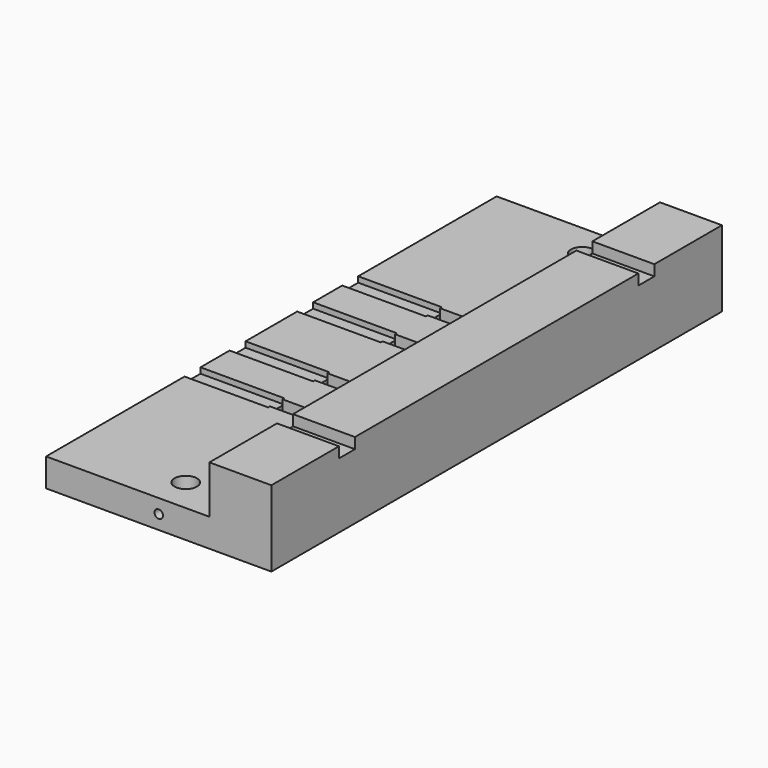
from build123d import *

# Parameters (mm, degrees)
F0_W     = 22
F0_H     = 30
F0_R     = 4
F0_R_2   = 1.5
F0_H_2   = 7.1
F0_H_3   = 125.8
F0_R_3   = 1.8
F1_DEPTH = 10
F2_DEPTH = 4.5
F3_DEPTH = 17
F4_DEPTH = 13.2
F5_R     = 1.5
F6_DEPTH = 15
F7_R     = 1.5
F8_DEPTH = 15
F9_DEPTH = 2


# Not quite as in the source:
# - a feature names something its author has since deleted; it is built from what else it names


with BuildPart() as f1:
    # F0 (on Top) → F1 (new body)
    with BuildSketch(Plane.XY):
        with Locations((29, -85)):
            Rectangle(F0_W, F0_H)
        with BuildLine():
            Line((-40, -100), (18, -100))
            Line((18, -100), (18, -70))
            Line((18, -70), (18, -62.9))
            Line((18, -62.9), (18, 62.9))
            Line((18, 62.9), (18, 70))
            Line((18, 70), (18, 100))
            Line((18, 100), (-40, 100))
            Line((-40, 100), (-40, 38.55))
            Line((-40, 38.55), (-10.3232520311, 38.55))
            Line((-10.3232520311, 38.55), (-10.3232520311, 37.75))
            Line((-10.3232520311, 37.75), (-2.3232520311, 37.75))
            ThreePointArc((-2.3232520311, 37.75), (3.6, 35), (-2.3232520311, 32.25))
            Line((-2.3232520311, 32.25), (-10.3232520311, 32.25))
            Line((-10.3232520311, 32.25), (-10.3232520311, 31.45))
            Line((-10.3232520311, 31.45), (-40, 31.45))
            Line((-40, 31.45), (-40, 18.55))
            Line((-40, 18.55), (-10.3232520311, 18.55))
            Line((-10.3232520311, 18.55), (-10.3232520311, 17.75))
            Line((-10.3232520311, 17.75), (-2.3232520311, 17.75))
            ThreePointArc((-2.3232520311, 17.75), (3.6, 15), (-2.3232520311, 12.25))
            Line((-2.3232520311, 12.25), (-10.3232520311, 12.25))
            Line((-10.3232520311, 12.25), (-10.3232520311, 11.45))
            Line((-10.3232520311, 11.45), (-40, 11.45))
            Line((-40, 11.45), (-40, -11.45))
            Line((-40, -11.45), (-10.3232520311, -11.45))
            Line((-10.3232520311, -11.45), (-10.3232520311, -12.25))
            Line((-10.3232520311, -12.25), (-2.3232520311, -12.25))
            ThreePointArc((-2.3232520311, -12.25), (3.6, -15), (-2.3232520311, -17.75))
            Line((-2.3232520311, -17.75), (-10.3232520311, -17.75))
            Line((-10.3232520311, -17.75), (-10.3232520311, -18.55))
            Line((-10.3232520311, -18.55), (-40, -18.55))
            Line((-40, -18.55), (-40, -31.45))
            Line((-40, -31.45), (-10.3232520311, -31.45))
            Line((-10.3232520311, -31.45), (-10.3232520311, -32.25))
            Line((-10.3232520311, -32.25), (-2.3232520311, -32.25))
            ThreePointArc((-2.3232520311, -32.25), (3.6, -35), (-2.3232520311, -37.75))
            Line((-2.3232520311, -37.75), (-10.3232520311, -37.75))
            Line((-10.3232520311, -37.75), (-10.3232520311, -38.55))
            Line((-10.3232520311, -38.55), (-40, -38.55))
            Line((-40, -38.55), (-40, -100))
        make_face()
        with Locations((0, -88)):
            Circle(F0_R, mode=Mode.SUBTRACT)
        with Locations((0, -66.45)):
            Circle(F0_R_2, mode=Mode.SUBTRACT)
        with Locations((0, 66.45)):
            Circle(F0_R_2, mode=Mode.SUBTRACT)
        with Locations((0, 88)):
            Circle(F0_R, mode=Mode.SUBTRACT)
        with Locations((29, -66.45)):
            Rectangle(F0_W, F0_H_2)
        with Locations((29, 0)):
            Rectangle(F0_W, F0_H_3)
        Polygon((-40, -31.45), (-40, -38.55), (-10.3232520311, -38.55), (-10.3232520311, -37.75), (-10.3232520311, -32.25), (-10.3232520311, -31.45), align=None)
        with Locations((29, 66.45)):
            Rectangle(F0_W, F0_H_2)
        with Locations((29, 85)):
            Rectangle(F0_W, F0_H)
        Polygon((-40, -11.45), (-40, -18.55), (-10.3232520311, -18.55), (-10.3232520311, -17.75), (-10.3232520311, -12.25), (-10.3232520311, -11.45), align=None)
        Polygon((-40, 18.55), (-40, 11.45), (-10.3232520311, 11.45), (-10.3232520311, 12.25), (-10.3232520311, 17.75), (-10.3232520311, 18.55), align=None)
        Polygon((-10.3232520311, 38.55), (-40, 38.55), (-40, 31.45), (-10.3232520311, 31.45), (-10.3232520311, 32.25), (-10.3232520311, 37.75), align=None)
        with BuildLine():
            Line((-10.3232520311, 17.75), (-10.3232520311, 12.25))
            Line((-10.3232520311, 12.25), (-2.3232520311, 12.25))
            ThreePointArc((-2.3232520311, 12.25), (3.6, 15), (-2.3232520311, 17.75))
            Line((-2.3232520311, 17.75), (-10.3232520311, 17.75))
        make_face()
        with Locations((0, 15)):
            Circle(F0_R_3, mode=Mode.SUBTRACT)
        with BuildLine():
            Line((-2.3232520311, 37.75), (-10.3232520311, 37.75))
            Line((-10.3232520311, 37.75), (-10.3232520311, 32.25))
            Line((-10.3232520311, 32.25), (-2.3232520311, 32.25))
            ThreePointArc((-2.3232520311, 32.25), (3.6, 35), (-2.3232520311, 37.75))
        make_face()
        with Locations((0, 35)):
            Circle(F0_R_3, mode=Mode.SUBTRACT)
        with BuildLine():
            Line((-10.3232520311, -12.25), (-10.3232520311, -17.75))
            Line((-10.3232520311, -17.75), (-2.3232520311, -17.75))
            ThreePointArc((-2.3232520311, -17.75), (3.6, -15), (-2.3232520311, -12.25))
            Line((-2.3232520311, -12.25), (-10.3232520311, -12.25))
        make_face()
        with Locations((0, -15)):
            Circle(F0_R_3, mode=Mode.SUBTRACT)
        with BuildLine():
            Line((-10.3232520311, -32.25), (-10.3232520311, -37.75))
            Line((-10.3232520311, -37.75), (-2.3232520311, -37.75))
            ThreePointArc((-2.3232520311, -37.75), (3.6, -35), (-2.3232520311, -32.25))
            Line((-2.3232520311, -32.25), (-10.3232520311, -32.25))
        make_face()
        with Locations((0, -35)):
            Circle(F0_R_3, mode=Mode.SUBTRACT)
    extrude(amount=-F1_DEPTH)

    # F0 (on Top) → F2 (cut)
    with BuildSketch(Plane.XY):
        with BuildLine():
            Line((-10.3232520311, -32.25), (-10.3232520311, -37.75))
            Line((-10.3232520311, -37.75), (-2.3232520311, -37.75))
            ThreePointArc((-2.3232520311, -37.75), (3.6, -35), (-2.3232520311, -32.25))
            Line((-2.3232520311, -32.25), (-10.3232520311, -32.25))
        make_face()
        with Locations((0, -35)):
            Circle(F0_R_3, mode=Mode.SUBTRACT)
        with BuildLine():
            Line((-10.3232520311, -12.25), (-10.3232520311, -17.75))
            Line((-10.3232520311, -17.75), (-2.3232520311, -17.75))
            ThreePointArc((-2.3232520311, -17.75), (3.6, -15), (-2.3232520311, -12.25))
            Line((-2.3232520311, -12.25), (-10.3232520311, -12.25))
        make_face()
        with Locations((0, -15)):
            Circle(F0_R_3, mode=Mode.SUBTRACT)
        with BuildLine():
            Line((-10.3232520311, 17.75), (-10.3232520311, 12.25))
            Line((-10.3232520311, 12.25), (-2.3232520311, 12.25))
            ThreePointArc((-2.3232520311, 12.25), (3.6, 15), (-2.3232520311, 17.75))
            Line((-2.3232520311, 17.75), (-10.3232520311, 17.75))
        make_face()
        with Locations((0, 15)):
            Circle(F0_R_3, mode=Mode.SUBTRACT)
        with BuildLine():
            Line((-2.3232520311, 37.75), (-10.3232520311, 37.75))
            Line((-10.3232520311, 37.75), (-10.3232520311, 32.25))
            Line((-10.3232520311, 32.25), (-2.3232520311, 32.25))
            ThreePointArc((-2.3232520311, 32.25), (3.6, 35), (-2.3232520311, 37.75))
        make_face()
        with Locations((0, 35)):
            Circle(F0_R_3, mode=Mode.SUBTRACT)
    extrude(amount=-F2_DEPTH, mode=Mode.SUBTRACT)

    # F0 (on Top) → F3 (join)
    with BuildSketch(Plane.XY):
        with Locations((29, -85)):
            Rectangle(F0_W, F0_H)
        with Locations((29, 85)):
            Rectangle(F0_W, F0_H)
        with Locations((29, 0)):
            Rectangle(F0_W, F0_H_3)
    extrude(amount=F3_DEPTH)

    # F0 (on Top) → F4 (join)
    with BuildSketch(Plane.XY):
        with Locations((29, 66.45)):
            Rectangle(F0_W, F0_H_2)
        with Locations((29, -66.45)):
            Rectangle(F0_W, F0_H_2)
    extrude(amount=F4_DEPTH)

    # F5 (on face) → F6 (cut)
    with BuildSketch(Plane(origin=(0, 100, 0), x_dir=(-1, 0, 0), z_dir=(0, 1, 0))):
        with Locations((0, -5)):
            Circle(F5_R)
    extrude(amount=-F6_DEPTH, mode=Mode.SUBTRACT)

    # F7 (on face) → F8 (cut)
    with BuildSketch(Plane.XZ.offset(100)):
        with Locations((0, -5)):
            Circle(F7_R)
    extrude(amount=-F8_DEPTH, mode=Mode.SUBTRACT)

    # F0 (on Top) → F9 (cut)
    with BuildSketch(Plane.XY):
        Polygon((-10.3232520311, 38.55), (-40, 38.55), (-40, 31.45), (-10.3232520311, 31.45), (-10.3232520311, 32.25), (-10.3232520311, 37.75), align=None)
        Polygon((-40, 18.55), (-40, 11.45), (-10.3232520311, 11.45), (-10.3232520311, 12.25), (-10.3232520311, 17.75), (-10.3232520311, 18.55), align=None)
        Polygon((-40, -11.45), (-40, -18.55), (-10.3232520311, -18.55), (-10.3232520311, -17.75), (-10.3232520311, -12.25), (-10.3232520311, -11.45), align=None)
        Polygon((-40, -31.45), (-40, -38.55), (-10.3232520311, -38.55), (-10.3232520311, -37.75), (-10.3232520311, -32.25), (-10.3232520311, -31.45), align=None)
    extrude(amount=-F9_DEPTH, mode=Mode.SUBTRACT)


solid = f1.part
